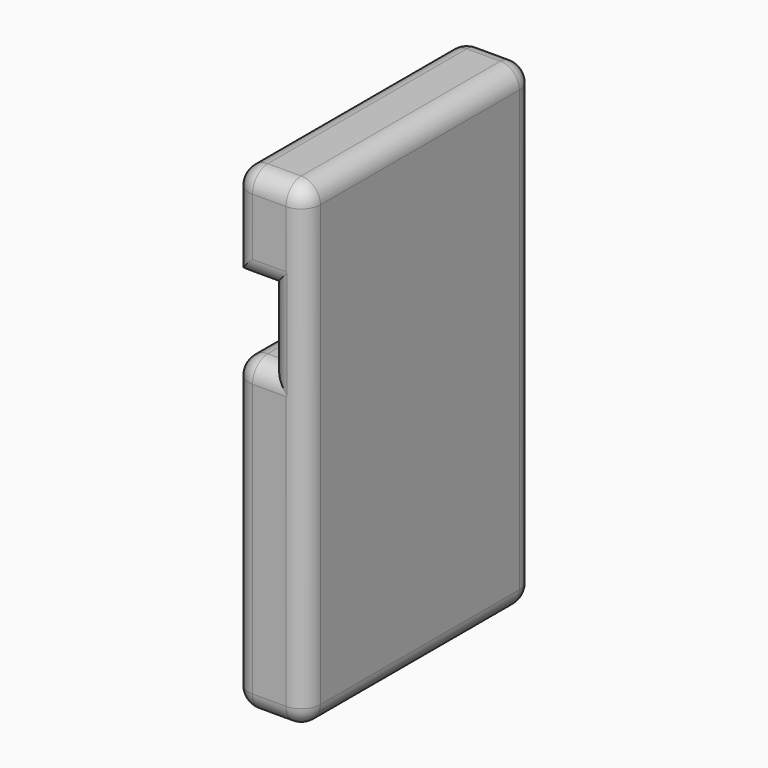
from build123d import *

# Parameters (mm, degrees)
F1_DEPTH      = 76.2
F2_T1_DEPTH   = 8.89
F2_T3_DEPTH   = 116.84
F2_T5_DEPTH   = 33.02
F2_T7_DEPTH   = 22.225
F2_T9_DEPTH   = 19.05
F2_T11_DEPTH  = 4.445
F2_T13_DEPTH  = 72.39
F2_T15_DEPTH  = 66.04
F2_S19_W      = 5.08
F2_S19_H      = 5.08
F2_T20_DEPTH  = 5.08
F2_S25_W      = 5.08
F2_S25_H      = 5.08
F2_T26_DEPTH  = 5.08
F2_S31_W      = 5.08
F2_S31_H      = 5.08
F2_T32_DEPTH  = 5.08
F2_S37_W      = 5.08
F2_S37_H      = 5.08
F2_T38_DEPTH  = 5.08
F2_S43_W      = 5.08
F2_S43_H      = 5.08
F2_T44_DEPTH  = 5.08
F2_S49_W      = 5.08
F2_S49_H      = 5.08
F2_T50_DEPTH  = 5.08
F2_S55_W      = 5.08
F2_S55_H      = 5.08
F2_T56_DEPTH  = 5.08
F2_S61_W      = 5.08
F2_S61_H      = 5.08
F2_T62_DEPTH  = 5.08
F2_S67_W      = 5.08
F2_S67_H      = 5.08
F2_T68_DEPTH  = 5.08
F2_S73_W      = 5.08
F2_S73_H      = 5.08
F2_T74_DEPTH  = 5.08
F2_T81_DEPTH  = 34.925
F2_T85_DEPTH  = 31.75
F2_T92_DEPTH  = 31.75
F2_T96_DEPTH  = 17.145
F2_T103_DEPTH = 34.925
F2_T107_DEPTH = 31.75
F2_T114_DEPTH = 31.75
F2_T118_DEPTH = 17.145
F3_T1_DEPTH   = 91.44


# Not quite as in the source:
# - a fillet or chamfer that OpenCascade refuses, or shapes differently, is made with other operations: its cross-section is extruded or revolved along the edge and cut away or added


with BuildPart() as f1:
    # F0 (on Front) → F1 (new body)
    with BuildSketch(Plane.XZ):
        Polygon((-19.05, -50.6151032805), (0, -50.6151032805), (0, 76.3848967195), (-19.05, 76.3848967195), (-19.05, 50.9848967195), (-9.525, 50.9848967195), (-9.525, 31.9348967195), (-19.05, 31.9348967195), align=None)
    extrude(amount=F1_DEPTH)

    # F2: fillet of radius 5.08 on 21 edges, made by hand

    # F2_s2 → F2_t1 (cut)
    with BuildSketch(Plane.YZ.offset(-13.97)):
        with BuildLine():
            ThreePointArc((-71.12, -50.6151032805), (-74.7121024484, -49.127205729), (-76.2, -45.5351032805))
            Line((-76.2, -45.5351032805), (-76.2, -50.6151032805))
            Line((-76.2, -50.6151032805), (-71.12, -50.6151032805))
        make_face()
        with BuildLine():
            ThreePointArc((-71.12, 76.3848967195), (-74.7121024484, 74.8969991679), (-76.2, 71.3048967195))
            Line((-76.2, 71.3048967195), (-76.2, 76.3848967195))
            Line((-76.2, 76.3848967195), (-71.12, 76.3848967195))
        make_face()
        with BuildLine():
            ThreePointArc((-5.08, 76.3848967195), (-1.4878975516, 74.8969991679), (0, 71.3048967195))
            Line((0, 71.3048967195), (0, 76.3848967195))
            Line((0, 76.3848967195), (-5.08, 76.3848967195))
        make_face()
        with BuildLine():
            ThreePointArc((-5.08, -50.6151032805), (-1.4878975516, -49.127205729), (0, -45.5351032805))
            Line((0, -45.5351032805), (0, -50.6151032805))
            Line((0, -50.6151032805), (-5.08, -50.6151032805))
        make_face()
    extrude(amount=F2_T1_DEPTH, mode=Mode.SUBTRACT)

    # F2_s4 → F2_t3 (cut)
    with BuildSketch(Plane.XY.offset(-45.5351032805)):
        with BuildLine():
            ThreePointArc((0, -71.12), (-1.4878975516, -74.7121024484), (-5.08, -76.2))
            Line((-5.08, -76.2), (0, -76.2))
            Line((0, -76.2), (0, -71.12))
        make_face()
        with BuildLine():
            ThreePointArc((0, -5.08), (-1.4878975516, -1.4878975516), (-5.08, 0))
            Line((-5.08, 0), (0, 0))
            Line((0, 0), (0, -5.08))
        make_face()
    extrude(amount=F2_T3_DEPTH, mode=Mode.SUBTRACT)

    # F2_s6 → F2_t5 (cut)
    with BuildSketch(Plane.XY.offset(38.2848967195)):
        with BuildLine():
            ThreePointArc((-19.05, -71.12), (-17.5621024484, -74.7121024484), (-13.97, -76.2))
            Line((-13.97, -76.2), (-19.05, -76.2))
            Line((-19.05, -76.2), (-19.05, -71.12))
        make_face()
        with BuildLine():
            ThreePointArc((-19.05, -5.08), (-17.5621024484, -1.4878975516), (-13.97, 0))
            Line((-13.97, 0), (-19.05, 0))
            Line((-19.05, 0), (-19.05, -5.08))
        make_face()
    extrude(amount=F2_T5_DEPTH, mode=Mode.SUBTRACT)

    # F2_s8 → F2_t7 (cut)
    with BuildSketch(Plane.YZ.offset(-31.75)):
        with BuildLine():
            ThreePointArc((-71.12, 50.9848967195), (-74.7121024484, 52.472794271), (-76.2, 56.0648967195))
            Line((-76.2, 56.0648967195), (-76.2, 50.9848967195))
            Line((-76.2, 50.9848967195), (-71.12, 50.9848967195))
        make_face()
        with BuildLine():
            ThreePointArc((-5.08, 50.9848967195), (-1.4878975516, 52.472794271), (0, 56.0648967195))
            Line((0, 56.0648967195), (0, 50.9848967195))
            Line((0, 50.9848967195), (-5.08, 50.9848967195))
        make_face()
    extrude(amount=F2_T7_DEPTH, mode=Mode.SUBTRACT)

    # F2_s10 → F2_t9 (cut)
    with BuildSketch(Plane.XY.offset(31.9348967195)):
        with BuildLine():
            ThreePointArc((-9.525, -71.12), (-8.0371024484, -74.7121024484), (-4.445, -76.2))
            Line((-4.445, -76.2), (-9.525, -76.2))
            Line((-9.525, -76.2), (-9.525, -71.12))
        make_face()
        with BuildLine():
            ThreePointArc((-9.525, -5.08), (-8.0371024484, -1.4878975516), (-4.445, 0))
            Line((-4.445, 0), (-9.525, 0))
            Line((-9.525, 0), (-9.525, -5.08))
        make_face()
    extrude(amount=F2_T9_DEPTH, mode=Mode.SUBTRACT)

    # F2_s12 → F2_t11 (cut)
    with BuildSketch(Plane.YZ.offset(-13.97)):
        with BuildLine():
            ThreePointArc((-71.12, 31.9348967195), (-74.7121024484, 30.4469991679), (-76.2, 26.8548967195))
            Line((-76.2, 26.8548967195), (-76.2, 31.9348967195))
            Line((-76.2, 31.9348967195), (-71.12, 31.9348967195))
        make_face()
        with BuildLine():
            ThreePointArc((-5.08, 31.9348967195), (-1.4878975516, 30.4469991679), (0, 26.8548967195))
            Line((0, 26.8548967195), (0, 31.9348967195))
            Line((0, 31.9348967195), (-5.08, 31.9348967195))
        make_face()
    extrude(amount=F2_T11_DEPTH, mode=Mode.SUBTRACT)

    # F2_s14 → F2_t13 (cut)
    with BuildSketch(Plane.XY.offset(-45.5351032805)):
        with BuildLine():
            ThreePointArc((-19.05, -71.12), (-17.5621024484, -74.7121024484), (-13.97, -76.2))
            Line((-13.97, -76.2), (-19.05, -76.2))
            Line((-19.05, -76.2), (-19.05, -71.12))
        make_face()
        with BuildLine():
            ThreePointArc((-19.05, -5.08), (-17.5621024484, -1.4878975516), (-13.97, 0))
            Line((-13.97, 0), (-19.05, 0))
            Line((-19.05, 0), (-19.05, -5.08))
        make_face()
    extrude(amount=F2_T13_DEPTH, mode=Mode.SUBTRACT)

    # F2_s16 → F2_t15 (cut)
    with BuildSketch(Plane.XZ.offset(5.08)):
        with BuildLine():
            ThreePointArc((0, 71.3048967195), (-1.4878975516, 74.8969991679), (-5.08, 76.3848967195))
            Line((-5.08, 76.3848967195), (0, 76.3848967195))
            Line((0, 76.3848967195), (0, 71.3048967195))
        make_face()
        with BuildLine():
            ThreePointArc((-13.97, 76.3848967195), (-17.5621024484, 74.8969991679), (-19.05, 71.3048967195))
            Line((-19.05, 71.3048967195), (-19.05, 76.3848967195))
            Line((-19.05, 76.3848967195), (-13.97, 76.3848967195))
        make_face()
        with BuildLine():
            ThreePointArc((-13.97, 31.9348967195), (-17.5621024484, 30.4469991679), (-19.05, 26.8548967195))
            Line((-19.05, 26.8548967195), (-19.05, 31.9348967195))
            Line((-19.05, 31.9348967195), (-13.97, 31.9348967195))
        make_face()
        with BuildLine():
            ThreePointArc((-13.97, -50.6151032805), (-17.5621024484, -49.127205729), (-19.05, -45.5351032805))
            Line((-19.05, -45.5351032805), (-19.05, -50.6151032805))
            Line((-19.05, -50.6151032805), (-13.97, -50.6151032805))
        make_face()
        with BuildLine():
            ThreePointArc((-5.08, -50.6151032805), (-1.4878975516, -49.127205729), (0, -45.5351032805))
            Line((0, -45.5351032805), (0, -50.6151032805))
            Line((0, -50.6151032805), (-5.08, -50.6151032805))
        make_face()
    extrude(amount=F2_T15_DEPTH, mode=Mode.SUBTRACT)


with BuildPart() as f2_tool18:
    # F2_s19 → F2_t20 (new body)
    with BuildSketch(Plane.XY.offset(-45.5351032805)):
        with Locations((-16.51, -73.66)):
            Rectangle(F2_S19_W, F2_S19_H)
    extrude(amount=-F2_T20_DEPTH)

    # F2_s21 → F2_t22 (revolve, cut)
    with BuildSketch(Plane(origin=(-13.97, -71.12, -45.5351032805), x_dir=(0.7071067812, 0.7071067812, 0), z_dir=(-0.7071067812, 0.7071067812, 0))):
        with BuildLine():
            ThreePointArc((0, -5.08), (5.08, 0), (0, 5.08))
            Line((0, 5.08), (0, -5.08))
        make_face()
    revolve(axis=Axis((-13.97, -71.12, -45.5351032805), (0, 0, -1)), mode=Mode.SUBTRACT)


with BuildPart() as f1_1:
    add(f1.part)

    # F2_t17: cut F2_tool18
    add(f2_tool18.part, mode=Mode.SUBTRACT)


with BuildPart() as f2_tool24:
    # F2_s25 → F2_t26 (new body)
    with BuildSketch(Plane.XY.offset(-45.5351032805)):
        with Locations((-2.54, -73.66)):
            Rectangle(F2_S25_W, F2_S25_H)
    extrude(amount=-F2_T26_DEPTH)

    # F2_s27 → F2_t28 (revolve, cut)
    with BuildSketch(Plane(origin=(-5.08, -71.12, -45.5351032805), x_dir=(-0.7071067812, 0.7071067812, 0), z_dir=(-0.7071067812, -0.7071067812, 0))):
        with BuildLine():
            ThreePointArc((0, -5.08), (5.08, 0), (0, 5.08))
            Line((0, 5.08), (0, -5.08))
        make_face()
    revolve(axis=Axis((-5.08, -71.12, -45.5351032805), (0, 0, -1)), mode=Mode.SUBTRACT)


with BuildPart() as f1_2:
    add(f1_1.part)

    # F2_t23: cut F2_tool24
    add(f2_tool24.part, mode=Mode.SUBTRACT)


with BuildPart() as f2_tool30:
    # F2_s31 → F2_t32 (new body)
    with BuildSketch(Plane.YZ.offset(-5.08)):
        with Locations((-73.66, 73.8448967195)):
            Rectangle(F2_S31_W, F2_S31_H)
    extrude(amount=F2_T32_DEPTH)

    # F2_s33 → F2_t34 (revolve, cut)
    with BuildSketch(Plane(origin=(-5.08, -71.12, 71.3048967195), x_dir=(0, 0.7071067812, -0.7071067812), z_dir=(0, -0.7071067812, -0.7071067812))):
        with BuildLine():
            ThreePointArc((0, -5.08), (5.08, 0), (0, 5.08))
            Line((0, 5.08), (0, -5.08))
        make_face()
    revolve(axis=Axis((-5.08, -71.12, 71.3048967195), (1, 0, 0)), mode=Mode.SUBTRACT)


with BuildPart() as f1_3:
    add(f1_2.part)

    # F2_t29: cut F2_tool30
    add(f2_tool30.part, mode=Mode.SUBTRACT)


with BuildPart() as f2_tool36:
    # F2_s37 → F2_t38 (new body)
    with BuildSketch(Plane.XZ.offset(71.12)):
        with Locations((-16.51, 73.8448967195)):
            Rectangle(F2_S37_W, F2_S37_H)
    extrude(amount=F2_T38_DEPTH)

    # F2_s39 → F2_t40 (revolve, cut)
    with BuildSketch(Plane(origin=(-13.97, -71.12, 71.3048967195), x_dir=(0.7071067812, 0, -0.7071067812), z_dir=(-0.7071067812, 0, -0.7071067812))):
        with BuildLine():
            ThreePointArc((0, -5.08), (5.08, 0), (0, 5.08))
            Line((0, 5.08), (0, -5.08))
        make_face()
    revolve(axis=Axis((-13.97, -71.12, 71.3048967195), (0, -1, 0)), mode=Mode.SUBTRACT)


with BuildPart() as f1_4:
    add(f1_3.part)

    # F2_t35: cut F2_tool36
    add(f2_tool36.part, mode=Mode.SUBTRACT)


with BuildPart() as f2_tool42:
    # F2_s43 → F2_t44 (new body)
    with BuildSketch(Plane.XZ.offset(71.12)):
        with Locations((-16.51, 29.3948967195)):
            Rectangle(F2_S43_W, F2_S43_H)
    extrude(amount=F2_T44_DEPTH)

    # F2_s45 → F2_t46 (revolve, cut)
    with BuildSketch(Plane(origin=(-13.97, -71.12, 26.8548967195), x_dir=(0.7071067812, 0, -0.7071067812), z_dir=(-0.7071067812, 0, -0.7071067812))):
        with BuildLine():
            ThreePointArc((0, -5.08), (5.08, 0), (0, 5.08))
            Line((0, 5.08), (0, -5.08))
        make_face()
    revolve(axis=Axis((-13.97, -71.12, 26.8548967195), (0, -1, 0)), mode=Mode.SUBTRACT)


with BuildPart() as f1_5:
    add(f1_4.part)

    # F2_t41: cut F2_tool42
    add(f2_tool42.part, mode=Mode.SUBTRACT)


with BuildPart() as f2_tool48:
    # F2_s49 → F2_t50 (new body)
    with BuildSketch(Plane.XZ.offset(5.08)):
        with Locations((-2.54, 73.8448967195)):
            Rectangle(F2_S49_W, F2_S49_H)
    extrude(amount=-F2_T50_DEPTH)

    # F2_s51 → F2_t52 (revolve, cut)
    with BuildSketch(Plane(origin=(-5.08, -5.08, 71.3048967195), x_dir=(-0.7071067812, 0, -0.7071067812), z_dir=(0.7071067812, 0, -0.7071067812))):
        with BuildLine():
            ThreePointArc((0, -5.08), (5.08, 0), (0, 5.08))
            Line((0, 5.08), (0, -5.08))
        make_face()
    revolve(axis=Axis((-5.08, -5.08, 71.3048967195), (0, 1, 0)), mode=Mode.SUBTRACT)


with BuildPart() as f1_6:
    add(f1_5.part)

    # F2_t47: cut F2_tool48
    add(f2_tool48.part, mode=Mode.SUBTRACT)


with BuildPart() as f2_tool54:
    # F2_s55 → F2_t56 (new body)
    with BuildSketch(Plane.XZ.offset(5.08)):
        with Locations((-16.51, 73.8448967195)):
            Rectangle(F2_S55_W, F2_S55_H)
    extrude(amount=-F2_T56_DEPTH)

    # F2_s57 → F2_t58 (revolve, cut)
    with BuildSketch(Plane(origin=(-13.97, -5.08, 71.3048967195), x_dir=(0.7071067812, 0, -0.7071067812), z_dir=(0.7071067812, 0, 0.7071067812))):
        with BuildLine():
            ThreePointArc((0, -5.08), (5.08, 0), (0, 5.08))
            Line((0, 5.08), (0, -5.08))
        make_face()
    revolve(axis=Axis((-13.97, -5.08, 71.3048967195), (0, 1, 0)), mode=Mode.SUBTRACT)


with BuildPart() as f1_7:
    add(f1_6.part)

    # F2_t53: cut F2_tool54
    add(f2_tool54.part, mode=Mode.SUBTRACT)


with BuildPart() as f2_tool60:
    # F2_s61 → F2_t62 (new body)
    with BuildSketch(Plane.XZ.offset(5.08)):
        with Locations((-16.51, 29.3948967195)):
            Rectangle(F2_S61_W, F2_S61_H)
    extrude(amount=-F2_T62_DEPTH)

    # F2_s63 → F2_t64 (revolve, cut)
    with BuildSketch(Plane(origin=(-13.97, -5.08, 26.8548967195), x_dir=(0.7071067812, 0, -0.7071067812), z_dir=(0.7071067812, 0, 0.7071067812))):
        with BuildLine():
            ThreePointArc((0, -5.08), (5.08, 0), (0, 5.08))
            Line((0, 5.08), (0, -5.08))
        make_face()
    revolve(axis=Axis((-13.97, -5.08, 26.8548967195), (0, 1, 0)), mode=Mode.SUBTRACT)


with BuildPart() as f1_8:
    add(f1_7.part)

    # F2_t59: cut F2_tool60
    add(f2_tool60.part, mode=Mode.SUBTRACT)


with BuildPart() as f2_tool66:
    # F2_s67 → F2_t68 (new body)
    with BuildSketch(Plane.XY.offset(-45.5351032805)):
        with Locations((-16.51, -2.54)):
            Rectangle(F2_S67_W, F2_S67_H)
    extrude(amount=-F2_T68_DEPTH)

    # F2_s69 → F2_t70 (revolve, cut)
    with BuildSketch(Plane(origin=(-13.97, -5.08, -45.5351032805), x_dir=(0.7071067812, -0.7071067812, 0), z_dir=(0.7071067812, 0.7071067812, 0))):
        with BuildLine():
            ThreePointArc((0, -5.08), (5.08, 0), (0, 5.08))
            Line((0, 5.08), (0, -5.08))
        make_face()
    revolve(axis=Axis((-13.97, -5.08, -45.5351032805), (0, 0, -1)), mode=Mode.SUBTRACT)


with BuildPart() as f1_9:
    add(f1_8.part)

    # F2_t65: cut F2_tool66
    add(f2_tool66.part, mode=Mode.SUBTRACT)


with BuildPart() as f2_tool72:
    # F2_s73 → F2_t74 (new body)
    with BuildSketch(Plane.XY.offset(-45.5351032805)):
        with Locations((-2.54, -2.54)):
            Rectangle(F2_S73_W, F2_S73_H)
    extrude(amount=-F2_T74_DEPTH)

    # F2_s75 → F2_t76 (revolve, cut)
    with BuildSketch(Plane(origin=(-5.08, -5.08, -45.5351032805), x_dir=(-0.7071067812, -0.7071067812, 0), z_dir=(0.7071067812, -0.7071067812, 0))):
        with BuildLine():
            ThreePointArc((0, -5.08), (5.08, 0), (0, 5.08))
            Line((0, 5.08), (0, -5.08))
        make_face()
    revolve(axis=Axis((-5.08, -5.08, -45.5351032805), (0, 0, -1)), mode=Mode.SUBTRACT)


with BuildPart() as f1_10:
    add(f1_9.part)

    # F2_t71: cut F2_tool72
    add(f2_tool72.part, mode=Mode.SUBTRACT)


with BuildPart() as f2_tool79:
    # F2_s80 → F2_t81 (new body)
    with BuildSketch(Plane.YZ.offset(-31.75)):
        with BuildLine():
            ThreePointArc((-71.12, 50.9848967195), (-74.7121024484, 52.472794271), (-76.2, 56.0648967195))
            Line((-76.2, 56.0648967195), (-76.2, 50.9848967195))
            Line((-76.2, 50.9848967195), (-71.12, 50.9848967195))
        make_face()
    extrude(amount=F2_T81_DEPTH)

    split(bisect_by=Plane.YZ.offset(-9.525), keep=Keep.TOP)


with BuildPart() as f2_tool83:
    # F2_s84 → F2_t85 (new body)
    with BuildSketch(Plane.XY.offset(63.6848967195)):
        with BuildLine():
            ThreePointArc((-9.525, -71.12), (-8.0371024484, -74.7121024484), (-4.445, -76.2))
            Line((-4.445, -76.2), (-9.525, -76.2))
            Line((-9.525, -76.2), (-9.525, -71.12))
        make_face()
    extrude(amount=-F2_T85_DEPTH)

    split(bisect_by=Plane.XY.offset(50.9848967195), keep=Keep.TOP)


with BuildPart() as f2_tool79_1:
    add(f2_tool79.part)

    # F2_t87: intersect F2_tool83
    add(f2_tool83.part, mode=Mode.INTERSECT)


with BuildPart() as f1_11:
    add(f1_10.part)

    # F2_t77: cut F2_tool79
    add(f2_tool79_1.part, mode=Mode.SUBTRACT)


with BuildPart() as f2_tool90:
    # F2_s91 → F2_t92 (new body)
    with BuildSketch(Plane.XY.offset(50.9848967195)):
        with BuildLine():
            ThreePointArc((-9.525, -71.12), (-8.0371024484, -74.7121024484), (-4.445, -76.2))
            Line((-4.445, -76.2), (-9.525, -76.2))
            Line((-9.525, -76.2), (-9.525, -71.12))
        make_face()
    extrude(amount=-F2_T92_DEPTH)

    split(bisect_by=Plane.XY.offset(31.9348967195), keep=Keep.BOTTOM)


with BuildPart() as f2_tool94:
    # F2_s95 → F2_t96 (new body)
    with BuildSketch(Plane.YZ.offset(3.175)):
        with BuildLine():
            ThreePointArc((-71.12, 31.9348967195), (-74.7121024484, 30.4469991679), (-76.2, 26.8548967195))
            Line((-76.2, 26.8548967195), (-76.2, 31.9348967195))
            Line((-76.2, 31.9348967195), (-71.12, 31.9348967195))
        make_face()
    extrude(amount=-F2_T96_DEPTH)

    split(bisect_by=Plane.YZ.offset(-9.525), keep=Keep.TOP)


with BuildPart() as f2_tool90_1:
    add(f2_tool90.part)

    # F2_t98: intersect F2_tool94
    add(f2_tool94.part, mode=Mode.INTERSECT)


with BuildPart() as f1_12:
    add(f1_11.part)

    # F2_t88: cut F2_tool90
    add(f2_tool90_1.part, mode=Mode.SUBTRACT)


with BuildPart() as f2_tool101:
    # F2_s102 → F2_t103 (new body)
    with BuildSketch(Plane.YZ.offset(-31.75)):
        with BuildLine():
            ThreePointArc((-5.08, 50.9848967195), (-1.4878975516, 52.472794271), (0, 56.0648967195))
            Line((0, 56.0648967195), (0, 50.9848967195))
            Line((0, 50.9848967195), (-5.08, 50.9848967195))
        make_face()
    extrude(amount=F2_T103_DEPTH)

    split(bisect_by=Plane.YZ.offset(-9.525), keep=Keep.TOP)


with BuildPart() as f2_tool105:
    # F2_s106 → F2_t107 (new body)
    with BuildSketch(Plane.XY.offset(63.6848967195)):
        with BuildLine():
            ThreePointArc((-9.525, -5.08), (-8.0371024484, -1.4878975516), (-4.445, 0))
            Line((-4.445, 0), (-9.525, 0))
            Line((-9.525, 0), (-9.525, -5.08))
        make_face()
    extrude(amount=-F2_T107_DEPTH)

    split(bisect_by=Plane.XY.offset(50.9848967195), keep=Keep.TOP)


with BuildPart() as f2_tool101_1:
    add(f2_tool101.part)

    # F2_t109: intersect F2_tool105
    add(f2_tool105.part, mode=Mode.INTERSECT)


with BuildPart() as f1_13:
    add(f1_12.part)

    # F2_t99: cut F2_tool101
    add(f2_tool101_1.part, mode=Mode.SUBTRACT)


with BuildPart() as f2_tool112:
    # F2_s113 → F2_t114 (new body)
    with BuildSketch(Plane.XY.offset(50.9848967195)):
        with BuildLine():
            ThreePointArc((-9.525, -5.08), (-8.0371024484, -1.4878975516), (-4.445, 0))
            Line((-4.445, 0), (-9.525, 0))
            Line((-9.525, 0), (-9.525, -5.08))
        make_face()
    extrude(amount=-F2_T114_DEPTH)

    split(bisect_by=Plane.XY.offset(31.9348967195), keep=Keep.BOTTOM)


with BuildPart() as f2_tool116:
    # F2_s117 → F2_t118 (new body)
    with BuildSketch(Plane.YZ.offset(3.175)):
        with BuildLine():
            ThreePointArc((-5.08, 31.9348967195), (-1.4878975516, 30.4469991679), (0, 26.8548967195))
            Line((0, 26.8548967195), (0, 31.9348967195))
            Line((0, 31.9348967195), (-5.08, 31.9348967195))
        make_face()
    extrude(amount=-F2_T118_DEPTH)

    split(bisect_by=Plane.YZ.offset(-9.525), keep=Keep.TOP)


with BuildPart() as f2_tool112_1:
    add(f2_tool112.part)

    # F2_t120: intersect F2_tool116
    add(f2_tool116.part, mode=Mode.INTERSECT)


with BuildPart() as f1_14:
    add(f1_13.part)

    # F2_t110: cut F2_tool112
    add(f2_tool112_1.part, mode=Mode.SUBTRACT)

    # F3: fillet of radius 5.08 on 4 edges, made by hand

    # F3_s2 → F3_t1 (cut)
    with BuildSketch(Plane.XZ.offset(-7.62)):
        with BuildLine():
            ThreePointArc((-19.05, 56.0648967195), (-17.5621024484, 52.472794271), (-13.97, 50.9848967195))
            Line((-13.97, 50.9848967195), (-19.05, 50.9848967195))
            Line((-19.05, 50.9848967195), (-19.05, 56.0648967195))
        make_face()
    extrude(amount=F3_T1_DEPTH, mode=Mode.SUBTRACT)


solid = f1_14.part
